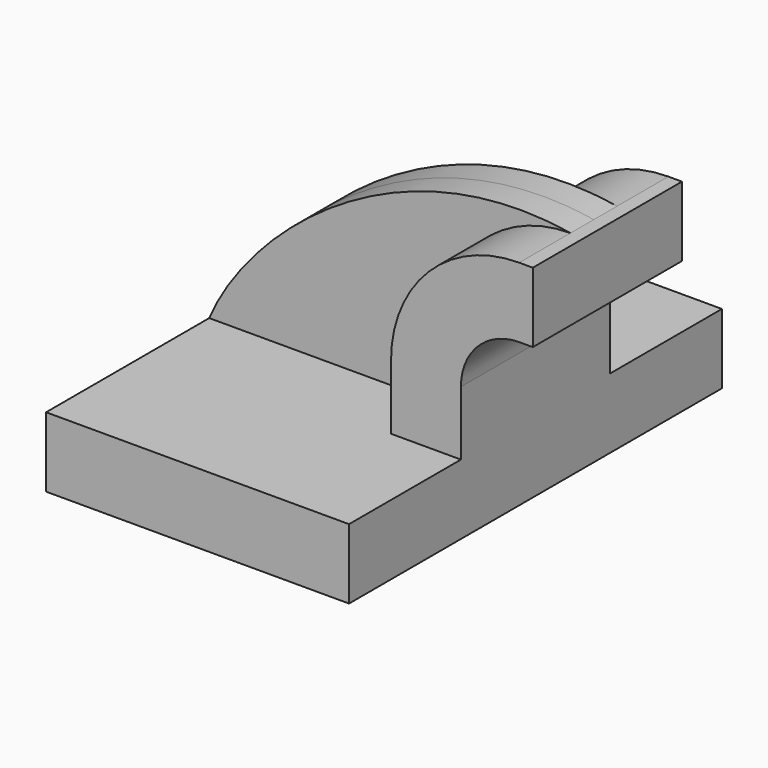
from build123d import *

# Parameters (mm, degrees)
F1_DEPTH = 63.5
F2_DEPTH = 25.4
F3_DEPTH = 7.9375


with BuildPart() as f1:
    # F0 (on Front) → F1 (new body, symmetric)
    with BuildSketch(Plane.XZ):
        Polygon((-41.275, 9.525), (-41.275, -9.525), (41.275, -9.525), (41.275, 9.525), (22.225, 9.525), align=None)
    extrude(amount=F1_DEPTH, both=True)

    # F0 (on Front) → F2 (join, symmetric)
    with BuildSketch(Plane.XZ):
        with BuildLine():
            Line((22.225, 9.525), (41.275, 9.525))
            Line((41.275, 9.525), (41.275, 27.0002))
            ThreePointArc((41.275, 27.0002), (45.9246798487, 38.2255201513), (57.15, 42.8752))
            Line((57.15, 42.8752), (60.8642640084, 42.8752))
            Line((60.8642640084, 42.8752), (60.8642640084, 61.9252))
            Line((60.8642640084, 61.9252), (57.15, 61.9252))
            ThreePointArc((57.15, 61.9252), (32.4542956671, 51.6959043329), (22.225, 27.0002))
            Line((22.225, 27.0002), (22.225, 9.525))
        make_face()
    extrude(amount=F2_DEPTH, both=True)

    # F0 (on Front) → F3 (join, symmetric)
    with BuildSketch(Plane.XZ):
        with BuildLine():
            add(Edge.make_bspline(
                [(-41.275, 9.525), (-30.5388011038, 34.9970385432), (9.5851859078, 69.7711631656), (57.15, 61.9252)],
                knots=[0, 0, 0, 0, 111.5045361635, 111.5045361635, 111.5045361635, 111.5045361635], degree=3))
            Line((-41.275, 9.525), (22.225, 9.525))
            Line((22.225, 9.525), (22.225, 27.0002))
            ThreePointArc((22.225, 27.0002), (32.4542956671, 51.6959043329), (57.15, 61.9252))
        make_face()
    extrude(amount=F3_DEPTH, both=True)


solid = f1.part
